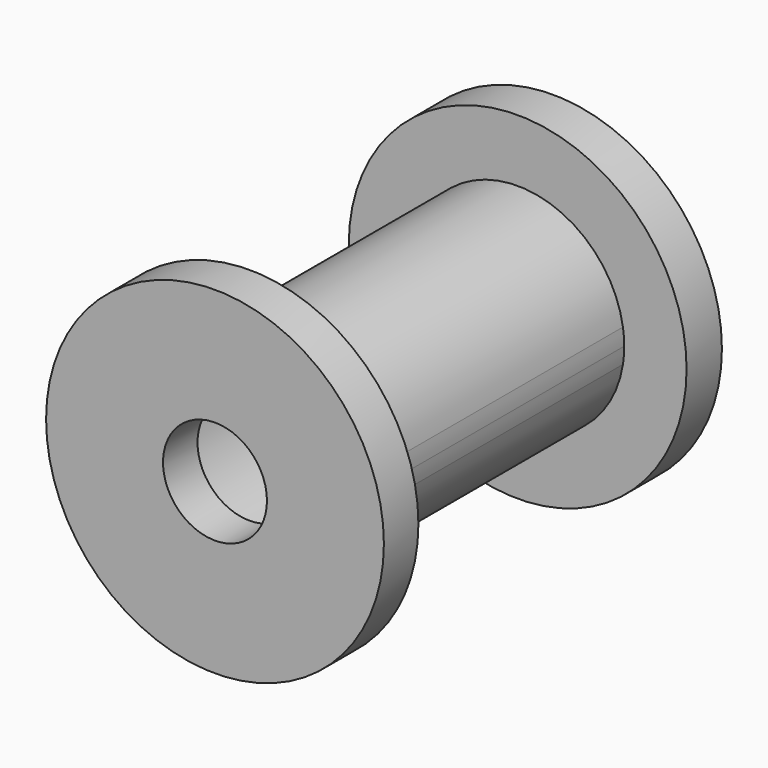
from build123d import *

# Parameters (mm, degrees)
F0_R     = 32.5
F0_R_2   = 10
F1_DEPTH = 81.3
F2_DEPTH = 7.2
F3_START = 8.5
F3_DEPTH = 64.5
F4_START = 8.5
F4_DEPTH = 64.5


with BuildPart() as f1:
    # F0 (on Front) → F1 (new body)
    with BuildSketch(Plane.XZ):
        Circle(F0_R)
        with BuildLine():
            ThreePointArc((-20.255, -3.159901106), (-22.25, 0), (-20.255, 3.159901106))
            ThreePointArc((-20.255, 3.159901106), (0, 20.5), (20.255, 3.159901106))
            ThreePointArc((20.255, 3.159901106), (21.7095185419, 1.8684886941), (22.25, 0))
            ThreePointArc((22.25, 0), (21.7095185419, -1.8684886941), (20.255, -3.159901106))
            ThreePointArc((20.255, -3.159901106), (0, -20.5), (-20.255, -3.159901106))
        make_face(mode=Mode.SUBTRACT)
        with BuildLine():
            ThreePointArc((-18.1750002352, 3.4524448251), (-16.0795600384, 2.2624655603), (-15.25, 0))
            ThreePointArc((-15.25, 0), (-16.0795600384, -2.2624655603), (-18.1750002352, -3.4524448251))
            ThreePointArc((-18.1750002352, -3.4524448251), (0, -18.5000002384), (18.1750002352, -3.4524448251))
            ThreePointArc((18.1750002352, -3.4524448251), (15.25, 0), (18.1750002352, 3.4524448251))
            ThreePointArc((18.1750002352, 3.4524448251), (0, 18.5000002384), (-18.1750002352, 3.4524448251))
        make_face()
        Circle(F0_R_2, mode=Mode.SUBTRACT)
        with BuildLine():
            ThreePointArc((-20.255, 3.159901106), (-19.2374633999, 3.4658879719), (-18.1750002352, 3.4524448251))
            ThreePointArc((-18.1750002352, 3.4524448251), (0, 18.5000002384), (18.1750002352, 3.4524448251))
            ThreePointArc((18.1750002352, 3.4524448251), (19.2374633999, 3.4658879719), (20.255, 3.159901106))
            ThreePointArc((20.255, 3.159901106), (0, 20.5), (-20.255, 3.159901106))
        make_face()
        with BuildLine():
            ThreePointArc((18.1750002352, -3.4524448251), (0, -18.5000002384), (-18.1750002352, -3.4524448251))
            ThreePointArc((-18.1750002352, -3.4524448251), (-19.2374633999, -3.4658879719), (-20.255, -3.159901106))
            ThreePointArc((-20.255, -3.159901106), (0, -20.5), (20.255, -3.159901106))
            ThreePointArc((20.255, -3.159901106), (19.2374633999, -3.4658879719), (18.1750002352, -3.4524448251))
        make_face()
        with BuildLine():
            ThreePointArc((-18.1750002352, -3.4524448251), (-16.0795600384, -2.2624655603), (-15.25, 0))
            ThreePointArc((-15.25, 0), (-16.0795600384, 2.2624655603), (-18.1750002352, 3.4524448251))
            ThreePointArc((-18.1750002352, 3.4524448251), (-18.5000002384, 0), (-18.1750002352, -3.4524448251))
        make_face()
        with BuildLine():
            ThreePointArc((18.5000002384, 0), (18.4185710291, 1.7338541081), (18.1750002352, 3.4524448251))
            ThreePointArc((18.1750002352, 3.4524448251), (15.25, 0), (18.1750002352, -3.4524448251))
            ThreePointArc((18.1750002352, -3.4524448251), (18.4185710291, -1.7338541081), (18.5000002384, 0))
        make_face()
        with BuildLine():
            ThreePointArc((20.255, 3.159901106), (19.2374633999, 3.4658879719), (18.1750002352, 3.4524448251))
            ThreePointArc((18.1750002352, 3.4524448251), (18.4185710291, 1.7338541081), (18.5000002384, 0))
            ThreePointArc((18.5000002384, 0), (18.4185710291, -1.7338541081), (18.1750002352, -3.4524448251))
            ThreePointArc((18.1750002352, -3.4524448251), (19.2374633999, -3.4658879719), (20.255, -3.159901106))
            ThreePointArc((20.255, -3.159901106), (20.4386582241, -1.5846923992), (20.5, 0))
            ThreePointArc((20.5, 0), (20.4386582241, 1.5846923992), (20.255, 3.159901106))
        make_face()
        with BuildLine():
            ThreePointArc((-18.1750002352, -3.4524448251), (-18.5000002384, 0), (-18.1750002352, 3.4524448251))
            ThreePointArc((-18.1750002352, 3.4524448251), (-19.2374633999, 3.4658879719), (-20.255, 3.159901106))
            ThreePointArc((-20.255, 3.159901106), (-20.5, 0), (-20.255, -3.159901106))
            ThreePointArc((-20.255, -3.159901106), (-19.2374633999, -3.4658879719), (-18.1750002352, -3.4524448251))
        make_face()
        with BuildLine():
            ThreePointArc((22.25, 0), (21.7095185419, 1.8684886941), (20.255, 3.159901106))
            ThreePointArc((20.255, 3.159901106), (20.4386582241, 1.5846923992), (20.5, 0))
            ThreePointArc((20.5, 0), (20.4386582241, -1.5846923992), (20.255, -3.159901106))
            ThreePointArc((20.255, -3.159901106), (21.7095185419, -1.8684886941), (22.25, 0))
        make_face()
        with BuildLine():
            ThreePointArc((-20.255, -3.159901106), (-20.5, 0), (-20.255, 3.159901106))
            ThreePointArc((-20.255, 3.159901106), (-22.25, 0), (-20.255, -3.159901106))
        make_face()
    extrude(amount=F1_DEPTH)

    # F0 (on Front) → F2 (cut)
    with BuildSketch(Plane.XZ):
        with BuildLine():
            ThreePointArc((22.25, 0), (21.7095185419, 1.8684886941), (20.255, 3.159901106))
            ThreePointArc((20.255, 3.159901106), (20.4386582241, 1.5846923992), (20.5, 0))
            ThreePointArc((20.5, 0), (20.4386582241, -1.5846923992), (20.255, -3.159901106))
            ThreePointArc((20.255, -3.159901106), (21.7095185419, -1.8684886941), (22.25, 0))
        make_face()
        with BuildLine():
            ThreePointArc((20.255, 3.159901106), (19.2374633999, 3.4658879719), (18.1750002352, 3.4524448251))
            ThreePointArc((18.1750002352, 3.4524448251), (18.4185710291, 1.7338541081), (18.5000002384, 0))
            ThreePointArc((18.5000002384, 0), (18.4185710291, -1.7338541081), (18.1750002352, -3.4524448251))
            ThreePointArc((18.1750002352, -3.4524448251), (19.2374633999, -3.4658879719), (20.255, -3.159901106))
            ThreePointArc((20.255, -3.159901106), (20.4386582241, -1.5846923992), (20.5, 0))
            ThreePointArc((20.5, 0), (20.4386582241, 1.5846923992), (20.255, 3.159901106))
        make_face()
        with BuildLine():
            ThreePointArc((-20.255, -3.159901106), (-20.5, 0), (-20.255, 3.159901106))
            ThreePointArc((-20.255, 3.159901106), (-22.25, 0), (-20.255, -3.159901106))
        make_face()
        with BuildLine():
            ThreePointArc((-18.1750002352, -3.4524448251), (-18.5000002384, 0), (-18.1750002352, 3.4524448251))
            ThreePointArc((-18.1750002352, 3.4524448251), (-19.2374633999, 3.4658879719), (-20.255, 3.159901106))
            ThreePointArc((-20.255, 3.159901106), (-20.5, 0), (-20.255, -3.159901106))
            ThreePointArc((-20.255, -3.159901106), (-19.2374633999, -3.4658879719), (-18.1750002352, -3.4524448251))
        make_face()
        with BuildLine():
            ThreePointArc((-18.1750002352, -3.4524448251), (-16.0795600384, -2.2624655603), (-15.25, 0))
            ThreePointArc((-15.25, 0), (-16.0795600384, 2.2624655603), (-18.1750002352, 3.4524448251))
            ThreePointArc((-18.1750002352, 3.4524448251), (-18.5000002384, 0), (-18.1750002352, -3.4524448251))
        make_face()
        with BuildLine():
            ThreePointArc((18.5000002384, 0), (18.4185710291, 1.7338541081), (18.1750002352, 3.4524448251))
            ThreePointArc((18.1750002352, 3.4524448251), (15.25, 0), (18.1750002352, -3.4524448251))
            ThreePointArc((18.1750002352, -3.4524448251), (18.4185710291, -1.7338541081), (18.5000002384, 0))
        make_face()
    extrude(amount=F2_DEPTH, mode=Mode.SUBTRACT)

    # F0 (on Front) → F3 (cut)
    with BuildSketch(Plane.XZ.offset(F3_START)):
        Circle(F0_R)
        with BuildLine():
            ThreePointArc((-20.255, -3.159901106), (-22.25, 0), (-20.255, 3.159901106))
            ThreePointArc((-20.255, 3.159901106), (0, 20.5), (20.255, 3.159901106))
            ThreePointArc((20.255, 3.159901106), (21.7095185419, 1.8684886941), (22.25, 0))
            ThreePointArc((22.25, 0), (21.7095185419, -1.8684886941), (20.255, -3.159901106))
            ThreePointArc((20.255, -3.159901106), (0, -20.5), (-20.255, -3.159901106))
        make_face(mode=Mode.SUBTRACT)
        with BuildLine():
            ThreePointArc((-20.255, -3.159901106), (-20.5, 0), (-20.255, 3.159901106))
            ThreePointArc((-20.255, 3.159901106), (-22.25, 0), (-20.255, -3.159901106))
        make_face()
        with BuildLine():
            ThreePointArc((22.25, 0), (21.7095185419, 1.8684886941), (20.255, 3.159901106))
            ThreePointArc((20.255, 3.159901106), (20.4386582241, 1.5846923992), (20.5, 0))
            ThreePointArc((20.5, 0), (20.4386582241, -1.5846923992), (20.255, -3.159901106))
            ThreePointArc((20.255, -3.159901106), (21.7095185419, -1.8684886941), (22.25, 0))
        make_face()
    extrude(amount=F3_DEPTH, mode=Mode.SUBTRACT)

    # F0 (on Front) → F4 (cut)
    with BuildSketch(Plane.XZ.offset(F4_START)):
        with BuildLine():
            ThreePointArc((-18.1750002352, 3.4524448251), (-16.0795600384, 2.2624655603), (-15.25, 0))
            ThreePointArc((-15.25, 0), (-16.0795600384, -2.2624655603), (-18.1750002352, -3.4524448251))
            ThreePointArc((-18.1750002352, -3.4524448251), (0, -18.5000002384), (18.1750002352, -3.4524448251))
            ThreePointArc((18.1750002352, -3.4524448251), (15.25, 0), (18.1750002352, 3.4524448251))
            ThreePointArc((18.1750002352, 3.4524448251), (0, 18.5000002384), (-18.1750002352, 3.4524448251))
        make_face()
        Circle(F0_R_2, mode=Mode.SUBTRACT)
        with BuildLine():
            ThreePointArc((-18.1750002352, -3.4524448251), (-16.0795600384, -2.2624655603), (-15.25, 0))
            ThreePointArc((-15.25, 0), (-16.0795600384, 2.2624655603), (-18.1750002352, 3.4524448251))
            ThreePointArc((-18.1750002352, 3.4524448251), (-18.5000002384, 0), (-18.1750002352, -3.4524448251))
        make_face()
        with BuildLine():
            ThreePointArc((18.5000002384, 0), (18.4185710291, 1.7338541081), (18.1750002352, 3.4524448251))
            ThreePointArc((18.1750002352, 3.4524448251), (15.25, 0), (18.1750002352, -3.4524448251))
            ThreePointArc((18.1750002352, -3.4524448251), (18.4185710291, -1.7338541081), (18.5000002384, 0))
        make_face()
    extrude(amount=F4_DEPTH, mode=Mode.SUBTRACT)


solid = f1.part
